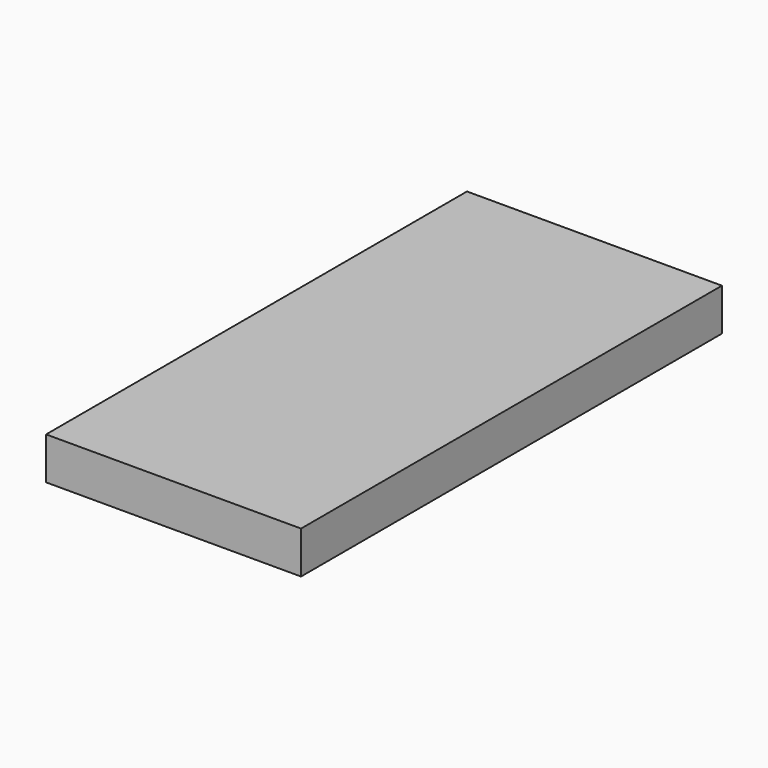
from build123d import *

# Parameters (mm, degrees)
F0_W     = 76.672680676
F0_H     = 158.2137197256
F1_DEPTH = 12.7


# Not quite as in the source:
# - the program builds the solid bodies; features that only make, move or delete a surface that nothing else refers to are left out


with BuildPart() as f1:
    # F0 (on Top) → F1 (new body)
    with BuildSketch(Plane.XY):
        with Locations((-38.336340338, 79.1068598628)):
            Rectangle(F0_W, F0_H)
    extrude(amount=F1_DEPTH)


solid = f1.part
